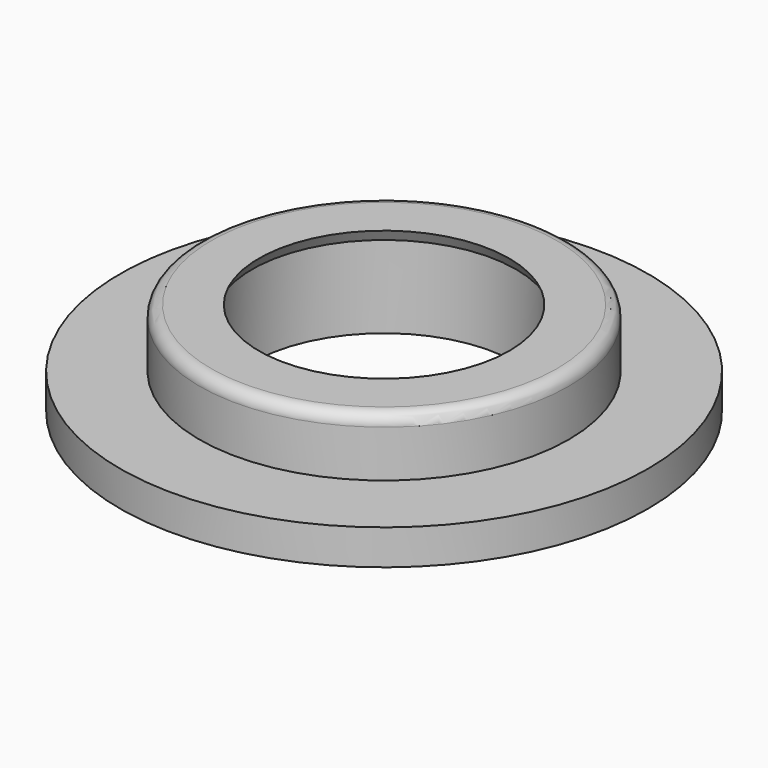
from build123d import *

# Parameters (mm, degrees)
F0_R        = 15.75
F0_R_2      = 11.25
F1_DEPTH    = 5
F2_R        = 22.5
F2_R_2      = 11.25
F3_DEPTH    = 3
F4_R        = 11.25
F4_R_2      = 10.25
F5_DEPTH    = 1
F6_S5_R     = 11.25
F6_T6_DEPTH = 17
F7_R        = 1


# Not quite as in the source:
# - a fillet or chamfer that OpenCascade refuses, or shapes differently, is made with other operations: its cross-section is extruded or revolved along the edge and cut away or added


with BuildPart() as f1:
    # F0 (on Top) → F1 (new body)
    with BuildSketch(Plane.XY):
        Circle(F0_R)
        Circle(F0_R_2, mode=Mode.SUBTRACT)
    extrude(amount=F1_DEPTH)

    # F2 (on face) → F3 (join)
    with BuildSketch(Plane(origin=(0, 0, 0), x_dir=(1, 0, 0), z_dir=(0, 0, -1))):
        Circle(F2_R)
        Circle(F2_R_2, mode=Mode.SUBTRACT)
    extrude(amount=F3_DEPTH)

    # F4 (on face) → F5 (join)
    with BuildSketch(Plane.XY.offset(5)):
        Circle(F4_R)
        Circle(F4_R_2, mode=Mode.SUBTRACT)
    extrude(amount=-F5_DEPTH)

    # F6: chamfer of 1 x 1.7320508076 on 1 edges, made by hand


with BuildPart() as f6_tool2:
    # F6_s3 → F6_t4 (revolve)
    with BuildSketch(Plane.XZ):
        Polygon((10.25, 5.7320508076), (11.25, 4), (10.25, 4), align=None)
    revolve(axis=Axis((0, 0, 4), (0, 0, 1)))

    # F6_s5 → F6_t6 (intersect, symmetric)
    with BuildSketch(Plane.XY.offset(4.9)):
        Circle(F6_S5_R)
    extrude(amount=F6_T6_DEPTH, both=True, mode=Mode.INTERSECT)


with BuildPart() as f1_1:
    add(f1.part)

    # F6_t1: cut F6_tool2
    add(f6_tool2.part, mode=Mode.SUBTRACT)

    # F7
    f7_edges = [f1_1.edges().sort_by_distance(p)[0] for p in [
        (-15.75, 0, 5),
    ]]
    fillet(f7_edges, radius=F7_R)


solid = f1_1.part
